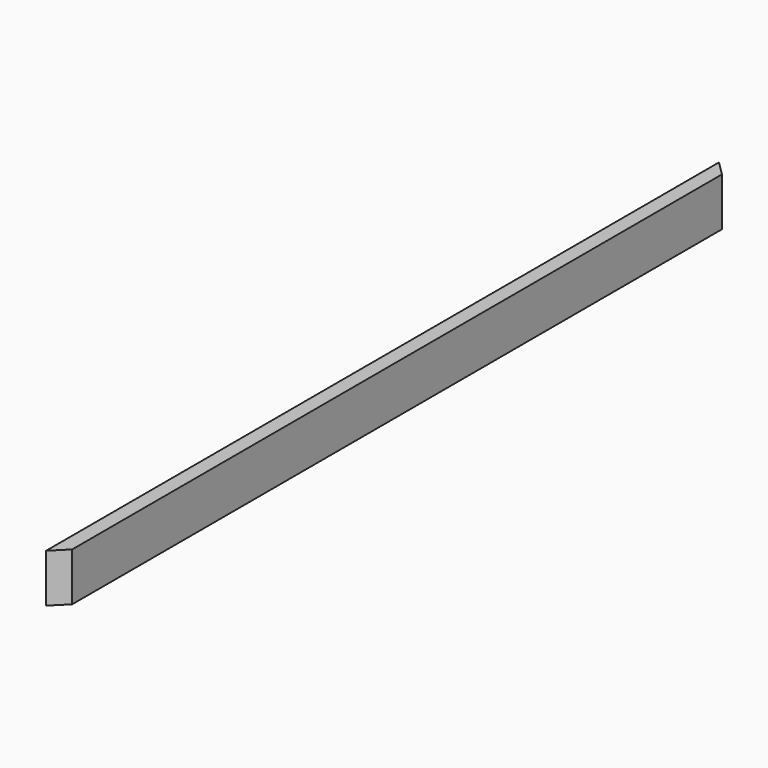
from build123d import *

# Parameters (mm, degrees)
F0_W     = 1104.9
F0_H     = 63.5
F1_DEPTH = 19.05
F2_SIZE  = 19.04999


# Not quite as in the source:
# - a fillet or chamfer is up to 0.001 mm smaller than in the source, because OpenCascade refuses the exact size


with BuildPart() as f1:
    # F0 (on Right) → F1 (new body)
    with BuildSketch(Plane.YZ):
        with Locations((-449.1316961765, -7.1268278062)):
            Rectangle(F0_W, F0_H)
    extrude(amount=F1_DEPTH)

    # F2 (size 19.05 in the source; OpenCascade refuses exactly that, so slightly less here)
    f2_edges = [f1.edges().sort_by_distance(p)[0] for p in [
        (19.05, -1001.581696, -7.126828),
        (19.05, 103.318304, -7.126828),
    ]]
    chamfer(f2_edges, length=F2_SIZE)


solid = f1.part
